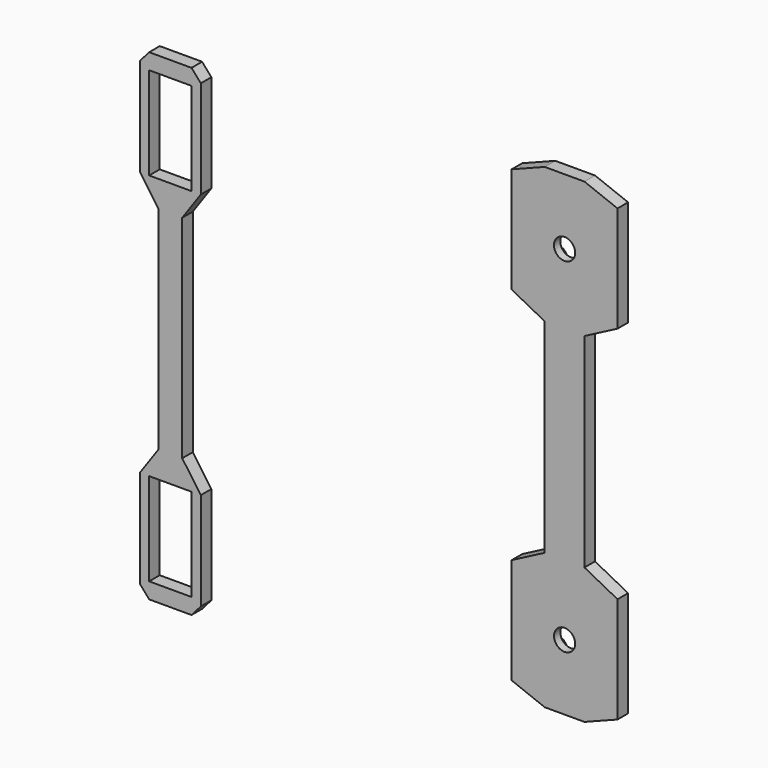
from build123d import *

# Parameters (mm, degrees)
F1_DEPTH = 6.35
F2_W     = 19.05
F2_H     = 8.2657442963
F2_H_2   = 48.8842557037
F3_DEPTH = 2.54
F4_R     = 5.08
F5_DEPTH = 3.81
F8_DEPTH = 3.81


# Not quite as in the source:
# - a feature names something its author has since deleted; it is built from what else it names


with BuildPart() as f1:
    # F0 (on Front) → F1 (new body)
    with BuildSketch(Plane.XZ):
        Polygon((-89.9882571208, 17.4341889973), (-85.5432571208, 17.4341889973), (-85.5432571208, 61.8841889973), (-65.2232571208, 61.8841889973), (-65.2232571208, 17.4341889973), (-60.7782571208, 17.4341889973), (-60.7782571208, 64.4241889973), (-89.9882571208, 64.4241889973), align=None)
        Polygon((-81.0982571208, 4.7341889973), (-81.0982571208, 17.4341889973), (-85.5432571208, 17.4341889973), (-89.9882571208, 17.4341889973), align=None)
        Polygon((-69.6682571208, 17.4341889973), (-81.0982571208, 17.4341889973), (-81.0982571208, 4.7341889973), (-81.0982571208, -46.0658110027), (-69.6682571208, -46.0658110027), (-69.6682571208, 4.7341889973), align=None)
        Polygon((-65.2232571208, 17.4341889973), (-69.6682571208, 17.4341889973), (-69.6682571208, 4.7341889973), (-60.7782571208, 17.4341889973), align=None)
        Polygon((-69.6682571208, -46.0658110027), (-81.0982571208, -46.0658110027), (-81.0982571208, -96.8658110027), (-81.0982571208, -109.5658110027), (-69.6682571208, -109.5658110027), (-69.6682571208, -96.8658110027), align=None)
        Polygon((-81.0982571208, -109.5658110027), (-81.0982571208, -96.8658110027), (-89.9882571208, -109.5658110027), (-85.5432571208, -109.5658110027), align=None)
        Polygon((-60.7782571208, -109.5658110027), (-69.6682571208, -96.8658110027), (-69.6682571208, -109.5658110027), (-65.2232571208, -109.5658110027), align=None)
        Polygon((-85.5432571208, -109.5658110027), (-89.9882571208, -109.5658110027), (-89.9882571208, -156.5558110027), (-60.7782571208, -156.5558110027), (-60.7782571208, -109.5658110027), (-65.2232571208, -109.5658110027), (-65.2232571208, -154.0158110027), (-85.5432571208, -154.0158110027), align=None)
        Polygon((-85.5432571208, 69.5041889973), (-89.9882571208, 64.4241889973), (-60.7782571208, 64.4241889973), (-65.2232571208, 69.5041889973), align=None)
        Polygon((-60.7782571208, -156.5558110027), (-89.9882571208, -156.5558110027), (-85.5432571208, -161.6358110027), (-65.2232571208, -161.6358110027), align=None)
    extrude(amount=F1_DEPTH)


with BuildPart() as f3:
    # F2 (on Front) → F3 (new body)
    with BuildSketch(Plane.XZ):
        Polygon((104.2609019141, -88.5054777617), (88.3859019141, -88.5054777617), (88.3859019141, -139.3054777617), (139.1859019141, -139.3054777617), (139.1859019141, -88.5054777617), (123.3109019141, -88.5054777617), align=None)
        with BuildLine():
            ThreePointArc((113.7859019141, -132.9554777617), (112.438863496, -132.3975161798), (111.8809019141, -131.0504777617))
            Line((111.8809019141, -131.0504777617), (109.4679019141, -119.5985076655))
            Line((109.4679019141, -119.5985076655), (108.0928720103, -118.2234777617))
            Line((108.0928720103, -118.2234777617), (96.6409019141, -115.8104777617))
            ThreePointArc((96.6409019141, -115.8104777617), (95.293863496, -115.2525161798), (94.7359019141, -113.9054777617))
            ThreePointArc((94.7359019141, -113.9054777617), (95.293863496, -112.5584393435), (96.6409019141, -112.0004777617))
            Line((96.6409019141, -112.0004777617), (108.0928720103, -109.5874777617))
            Line((108.0928720103, -109.5874777617), (109.4679019141, -108.2124478579))
            Line((109.4679019141, -108.2124478579), (111.8809019141, -96.7604777617))
            ThreePointArc((111.8809019141, -96.7604777617), (112.438863496, -95.4134393435), (113.7859019141, -94.8554777617))
            ThreePointArc((113.7859019141, -94.8554777617), (115.1329403323, -95.4134393435), (115.6909019141, -96.7604777617))
            Line((115.6909019141, -96.7604777617), (118.1039019141, -108.2124478579))
            Line((118.1039019141, -108.2124478579), (119.4789318179, -109.5874777617))
            Line((119.4789318179, -109.5874777617), (130.9309019141, -112.0004777617))
            ThreePointArc((130.9309019141, -112.0004777617), (132.2779403323, -112.5584393435), (132.8359019141, -113.9054777617))
            ThreePointArc((132.8359019141, -113.9054777617), (132.2779403323, -115.2525161798), (130.9309019141, -115.8104777617))
            Line((130.9309019141, -115.8104777617), (119.4789318179, -118.2234777617))
            Line((119.4789318179, -118.2234777617), (118.1039019141, -119.5985076655))
            Line((118.1039019141, -119.5985076655), (115.6909019141, -131.0504777617))
            ThreePointArc((115.6909019141, -131.0504777617), (115.1329403323, -132.3975161798), (113.7859019141, -132.9554777617))
        make_face(mode=Mode.SUBTRACT)
        Polygon((139.1859019141, -139.3054777617), (88.3859019141, -139.3054777617), (104.2609019141, -145.4785017002), (123.3109019141, -145.4785017002), align=None)
        Polygon((104.2609019141, -88.5054777617), (104.2609019141, -80.2397334654), (88.3859019141, -88.5054777617), align=None)
        with Locations((113.7859019141, -84.3726056135)):
            Rectangle(F2_W, F2_H)
        Polygon((139.1859019141, -88.5054777617), (123.3109019141, -80.2397334654), (123.3109019141, -88.5054777617), align=None)
        with Locations((113.7859019141, -55.7976056135)):
            Rectangle(F2_W, F2_H_2)
        with Locations((113.7859019141, -6.9133499098)):
            Rectangle(F2_W, F2_H_2)
        Polygon((139.1859019141, 76.5945222383), (88.3859019141, 76.5945222383), (88.3859019141, 25.7945222383), (104.2609019141, 25.7945222383), (123.3109019141, 25.7945222383), (139.1859019141, 25.7945222383), align=None)
        with BuildLine():
            Line((109.4679019141, 56.8875521421), (111.8809019141, 68.3395222383))
            ThreePointArc((111.8809019141, 68.3395222383), (112.438863496, 69.6865606565), (113.7859019141, 70.2445222383))
            ThreePointArc((113.7859019141, 70.2445222383), (115.1329403323, 69.6865606565), (115.6909019141, 68.3395222383))
            Line((115.6909019141, 68.3395222383), (118.1039019141, 56.8875521421))
            Line((118.1039019141, 56.8875521421), (119.4789318179, 55.5125222383))
            Line((119.4789318179, 55.5125222383), (130.9309019141, 53.0995222383))
            ThreePointArc((130.9309019141, 53.0995222383), (132.2779403323, 52.5415606565), (132.8359019141, 51.1945222383))
            ThreePointArc((132.8359019141, 51.1945222383), (132.2779403323, 49.8474838202), (130.9309019141, 49.2895222383))
            Line((130.9309019141, 49.2895222383), (119.4789318179, 46.8765222383))
            Line((119.4789318179, 46.8765222383), (118.1039019141, 45.5014923345))
            Line((118.1039019141, 45.5014923345), (115.6909019141, 34.0495222383))
            ThreePointArc((115.6909019141, 34.0495222383), (115.1329403323, 32.7024838202), (113.7859019141, 32.1445222383))
            ThreePointArc((113.7859019141, 32.1445222383), (112.438863496, 32.7024838202), (111.8809019141, 34.0495222383))
            Line((111.8809019141, 34.0495222383), (109.4679019141, 45.5014923345))
            Line((109.4679019141, 45.5014923345), (108.0928720103, 46.8765222383))
            Line((108.0928720103, 46.8765222383), (96.6409019141, 49.2895222383))
            ThreePointArc((96.6409019141, 49.2895222383), (95.293863496, 49.8474838202), (94.7359019141, 51.1945222383))
            ThreePointArc((94.7359019141, 51.1945222383), (95.293863496, 52.5415606565), (96.6409019141, 53.0995222383))
            Line((96.6409019141, 53.0995222383), (108.0928720103, 55.5125222383))
            Line((108.0928720103, 55.5125222383), (109.4679019141, 56.8875521421))
        make_face(mode=Mode.SUBTRACT)
        Polygon((104.2609019141, 25.7945222383), (88.3859019141, 25.7945222383), (104.2609019141, 17.5287779421), align=None)
        with Locations((113.7859019141, 21.6616500902)):
            Rectangle(F2_W, F2_H)
        Polygon((123.3109019141, 17.5287779421), (139.1859019141, 25.7945222383), (123.3109019141, 25.7945222383), align=None)
        Polygon((104.2609019141, 82.7675461769), (88.3859019141, 76.5945222383), (139.1859019141, 76.5945222383), (123.3109019141, 82.7675461769), align=None)
    extrude(amount=F3_DEPTH)

    # F4 (on face) → F5 (join)
    with BuildSketch(Plane.XZ.offset(2.54)):
        Polygon((104.2609019141, -31.3554777617), (123.3109019141, -31.3554777617), (123.3109019141, 17.5287779421), (139.1859019141, 25.7945222383), (139.1859019141, 76.5945222383), (123.3109019141, 82.7675461769), (104.2609019141, 82.7675461769), (88.3859019141, 76.5945222383), (88.3859019141, 25.7945222383), (104.2609019141, 17.5287779421), align=None)
        with BuildLine():
            Line((108.0928720103, 55.5125222383), (109.4679019141, 56.8875521421))
            Line((109.4679019141, 56.8875521421), (111.8809019141, 68.3395222383))
            ThreePointArc((111.8809019141, 68.3395222383), (113.7859019141, 70.2445222383), (115.6909019141, 68.3395222383))
            Line((115.6909019141, 68.3395222383), (118.1039019141, 56.8875521421))
            Line((118.1039019141, 56.8875521421), (119.4789318179, 55.5125222383))
            Line((119.4789318179, 55.5125222383), (130.9309019141, 53.0995222383))
            ThreePointArc((130.9309019141, 53.0995222383), (132.8359019141, 51.1945222383), (130.9309019141, 49.2895222383))
            Line((130.9309019141, 49.2895222383), (119.4789318179, 46.8765222383))
            Line((119.4789318179, 46.8765222383), (118.1039019141, 45.5014923345))
            Line((118.1039019141, 45.5014923345), (115.6909019141, 34.0495222383))
            ThreePointArc((115.6909019141, 34.0495222383), (113.7859019141, 32.1445222383), (111.8809019141, 34.0495222383))
            Line((111.8809019141, 34.0495222383), (109.4679019141, 45.5014923345))
            Line((109.4679019141, 45.5014923345), (108.0928720103, 46.8765222383))
            Line((108.0928720103, 46.8765222383), (96.6409019141, 49.2895222383))
            ThreePointArc((96.6409019141, 49.2895222383), (94.7359019141, 51.1945222383), (96.6409019141, 53.0995222383))
            Line((96.6409019141, 53.0995222383), (108.0928720103, 55.5125222383))
        make_face(mode=Mode.SUBTRACT)
        with BuildLine():
            Line((111.8809019141, 68.3395222383), (109.4679019141, 56.8875521421))
            Line((109.4679019141, 56.8875521421), (108.0928720103, 55.5125222383))
            Line((108.0928720103, 55.5125222383), (96.6409019141, 53.0995222383))
            ThreePointArc((96.6409019141, 53.0995222383), (94.7359019141, 51.1945222383), (96.6409019141, 49.2895222383))
            Line((96.6409019141, 49.2895222383), (108.0928720103, 46.8765222383))
            Line((108.0928720103, 46.8765222383), (109.4679019141, 45.5014923345))
            Line((109.4679019141, 45.5014923345), (111.8809019141, 34.0495222383))
            ThreePointArc((111.8809019141, 34.0495222383), (113.7859019141, 32.1445222383), (115.6909019141, 34.0495222383))
            Line((115.6909019141, 34.0495222383), (118.1039019141, 45.5014923345))
            Line((118.1039019141, 45.5014923345), (119.4789318179, 46.8765222383))
            Line((119.4789318179, 46.8765222383), (130.9309019141, 49.2895222383))
            ThreePointArc((130.9309019141, 49.2895222383), (132.8359019141, 51.1945222383), (130.9309019141, 53.0995222383))
            Line((130.9309019141, 53.0995222383), (119.4789318179, 55.5125222383))
            Line((119.4789318179, 55.5125222383), (118.1039019141, 56.8875521421))
            Line((118.1039019141, 56.8875521421), (115.6909019141, 68.3395222383))
            ThreePointArc((115.6909019141, 68.3395222383), (113.7859019141, 70.2445222383), (111.8809019141, 68.3395222383))
        make_face()
        with Locations((113.7798130512, 51.2091144919)):
            Circle(F4_R, mode=Mode.SUBTRACT)
    extrude(amount=F5_DEPTH)

    # F4 (on face) → F8 (join)
    with BuildSketch(Plane.XZ.offset(2.54)):
        Polygon((123.3109019141, -80.2397334654), (123.3109019141, -31.3554777617), (104.2609019141, -31.3554777617), (104.2609019141, -80.2397334654), (88.3859019141, -88.5054777617), (88.3859019141, -139.3054777617), (104.2609019141, -145.4785017002), (123.3109019141, -145.4785017002), (139.1859019141, -139.3054777617), (139.1859019141, -88.5054777617), align=None)
        with BuildLine():
            ThreePointArc((130.9309019141, -112.0004777617), (132.8359019141, -113.9054777617), (130.9309019141, -115.8104777617))
            Line((130.9309019141, -115.8104777617), (119.4789318179, -118.2234777617))
            Line((119.4789318179, -118.2234777617), (118.1039019141, -119.5985076655))
            Line((118.1039019141, -119.5985076655), (115.6909019141, -131.0504777617))
            ThreePointArc((115.6909019141, -131.0504777617), (113.7859019141, -132.9554777617), (111.8809019141, -131.0504777617))
            Line((111.8809019141, -131.0504777617), (109.4679019141, -119.5985076655))
            Line((109.4679019141, -119.5985076655), (108.0928720103, -118.2234777617))
            Line((108.0928720103, -118.2234777617), (96.6409019141, -115.8104777617))
            ThreePointArc((96.6409019141, -115.8104777617), (94.7359019141, -113.9054777617), (96.6409019141, -112.0004777617))
            Line((96.6409019141, -112.0004777617), (108.0928720103, -109.5874777617))
            Line((108.0928720103, -109.5874777617), (109.4679019141, -108.2124478579))
            Line((109.4679019141, -108.2124478579), (111.8809019141, -96.7604777617))
            ThreePointArc((111.8809019141, -96.7604777617), (113.7859019141, -94.8554777617), (115.6909019141, -96.7604777617))
            Line((115.6909019141, -96.7604777617), (118.1039019141, -108.2124478579))
            Line((118.1039019141, -108.2124478579), (119.4789318179, -109.5874777617))
            Line((119.4789318179, -109.5874777617), (130.9309019141, -112.0004777617))
        make_face(mode=Mode.SUBTRACT)
        with BuildLine():
            Line((119.4789318179, -118.2234777617), (130.9309019141, -115.8104777617))
            ThreePointArc((130.9309019141, -115.8104777617), (132.8359019141, -113.9054777617), (130.9309019141, -112.0004777617))
            Line((130.9309019141, -112.0004777617), (119.4789318179, -109.5874777617))
            Line((119.4789318179, -109.5874777617), (118.1039019141, -108.2124478579))
            Line((118.1039019141, -108.2124478579), (115.6909019141, -96.7604777617))
            ThreePointArc((115.6909019141, -96.7604777617), (113.7859019141, -94.8554777617), (111.8809019141, -96.7604777617))
            Line((111.8809019141, -96.7604777617), (109.4679019141, -108.2124478579))
            Line((109.4679019141, -108.2124478579), (108.0928720103, -109.5874777617))
            Line((108.0928720103, -109.5874777617), (96.6409019141, -112.0004777617))
            ThreePointArc((96.6409019141, -112.0004777617), (94.7359019141, -113.9054777617), (96.6409019141, -115.8104777617))
            Line((96.6409019141, -115.8104777617), (108.0928720103, -118.2234777617))
            Line((108.0928720103, -118.2234777617), (109.4679019141, -119.5985076655))
            Line((109.4679019141, -119.5985076655), (111.8809019141, -131.0504777617))
            ThreePointArc((111.8809019141, -131.0504777617), (113.7859019141, -132.9554777617), (115.6909019141, -131.0504777617))
            Line((115.6909019141, -131.0504777617), (118.1039019141, -119.5985076655))
            Line((118.1039019141, -119.5985076655), (119.4789318179, -118.2234777617))
        make_face()
        with Locations((113.7798130512, -113.9200700153)):
            Circle(F4_R, mode=Mode.SUBTRACT)
    extrude(amount=F8_DEPTH)


solid = Compound([f1.part, f3.part])
